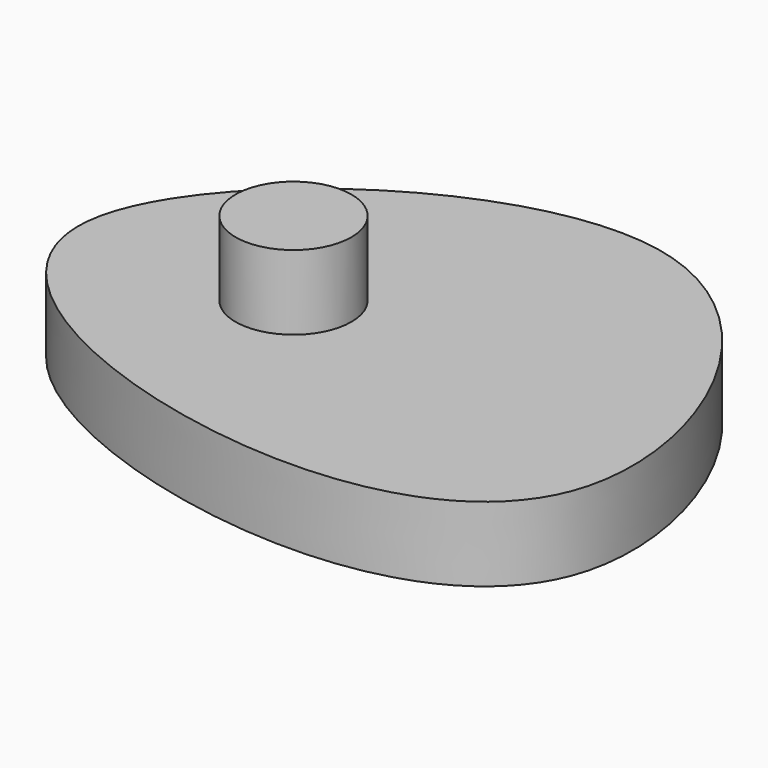
from build123d import *

# Parameters (mm, degrees)
F1_DEPTH = 25.4
F2_R     = 19.7424268159
F3_DEPTH = 25.4


with BuildPart() as f1:
    # F0 (on Top) → F1 (new body)
    with BuildSketch(Plane.XY):
        with BuildLine():
            add(Edge.make_bspline(
                [(-97.1121788025, 20.6361096352), (-93.0276525884, 61.9393701555), (51.4956922911, 165.1047163075), (140.5592801262, -42.1156070839), (-0.8499035212, -69.1319386587), (-100.7330246446, -15.9783546332), (-97.1121788025, 20.6361096352)],
                knots=[0, 0, 0, 0, 0.2728617823, 0.5310717847, 0.7581138183, 1, 1, 1, 1], degree=3))
        make_face()
    extrude(amount=F1_DEPTH)

    # F2 (on face) → F3 (join)
    with BuildSketch(Plane.XY.offset(25.4)):
        with Locations((-25.7869306952, 19.2524194717)):
            Circle(F2_R)
    extrude(amount=F3_DEPTH)


solid = f1.part
